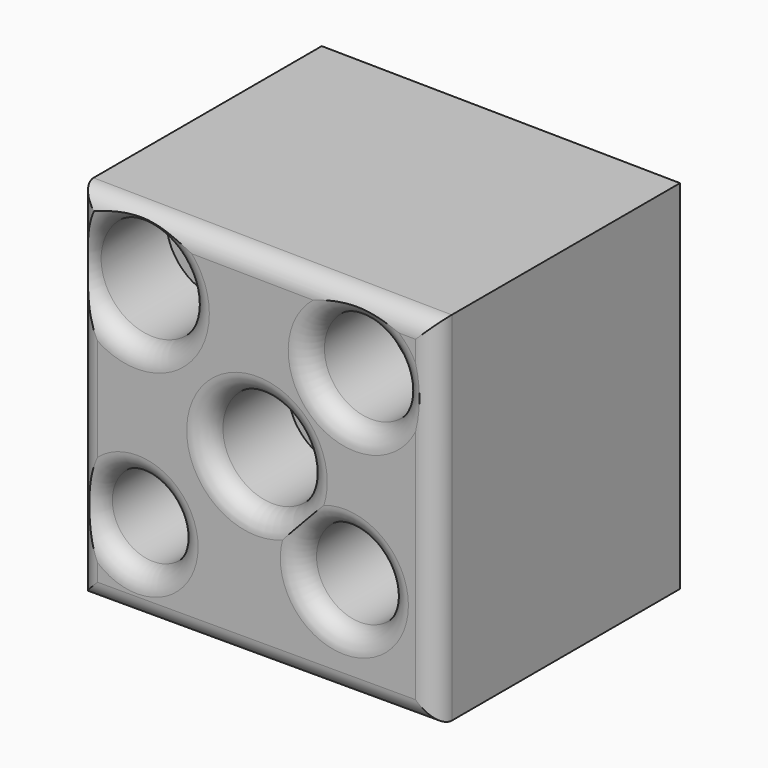
from build123d import *

# Parameters (mm, degrees)
F1_DEPTH    = 76.2
F2_R        = 13.0009566934
F2_R_2      = 11.7691858669
F2_R_3      = 12.5140273394
F2_R_4      = 10.2035026267
F2_R_5      = 10.9635179416
F4_DEPTH    = 25.4
F5_T1_DEPTH = 114.7959034965
F5_T3_DEPTH = 114.5331439546
F5_T5_DEPTH = 115.5605603925
F5_T7_DEPTH = 114.7899989954


# Not quite as in the source:
# - a fillet or chamfer that OpenCascade refuses, or shapes differently, is made with other operations: its cross-section is extruded or revolved along the edge and cut away or added


with BuildPart() as f1:
    # F0 (on Front) → F1 (new body)
    with BuildSketch(Plane.XZ):
        Polygon((56.2510117888, 48.6738197505), (-33.1341587007, 49.7012361884), (-33.1341587007, -40.4544956982), (56.2510117888, -40.4544956982), align=None)
    extrude(amount=F1_DEPTH)

    # F2 (on face) → F4 (cut)
    with BuildSketch(Plane.XZ.offset(76.2)):
        with Locations((-18.2341039181, 32.6071083546)):
            Circle(F2_R)
        with Locations((36.246843636, 30.9728365391)):
            Circle(F2_R_2)
        with Locations((11.6678411141, 5.1815295592)):
            Circle(F2_R_3)
        with Locations((-18.2341039181, -19.5480342954)):
            Circle(F2_R_4)
        with Locations((33.4707759321, -15.3220649809)):
            Circle(F2_R_5)
    extrude(amount=-F4_DEPTH, mode=Mode.SUBTRACT)

    # F5: fillet of radius 5.08 on 9 edges, made by hand

    # F5_s2 → F5_t1 (cut)
    with BuildSketch(Plane(origin=(68.3857605657, 0, -0.7860437491), x_dir=(0, 1, 0), z_dir=(-0.9999339475, 0, 0.0114935013))):
        with BuildLine():
            ThreePointArc((-71.1190343146, -49.3175258025), (-74.7121024484, -47.829228251), (-76.2004, -44.2361601171))
            Line((-76.2004, -44.2361601171), (-76.7085365685, -44.2361601171))
            ThreePointArc((-76.7085365685, -44.2361601171), (-76.7081365685, -46.7766429598), (-76.7081365685, -49.3171258025))
            Line((-76.7081365685, -49.3171258025), (-76.2, -49.8252623711))
            ThreePointArc((-76.2, -49.8252623711), (-73.6595171573, -49.8252623711), (-71.1190343146, -49.8256623711))
            Line((-71.1190343146, -49.8256623711), (-71.1190343146, -49.3175258025))
        make_face()
    extrude(amount=F5_T1_DEPTH, mode=Mode.SUBTRACT)

    # F5_s4 → F5_t3 (cut)
    with BuildSketch(Plane.XY.offset(-53.1569099511)):
        with BuildLine():
            ThreePointArc((56.2514117888, -71.1190343146), (54.7631142373, -74.7121024484), (51.1700461034, -76.2004))
            Line((51.1700461034, -76.2004), (51.1700461034, -76.7085365685))
            ThreePointArc((51.1700461034, -76.7085365685), (53.7105289461, -76.7081365685), (56.2510117888, -76.7081365685))
            Line((56.2510117888, -76.7081365685), (56.7591483574, -76.2))
            ThreePointArc((56.7591483574, -76.2), (56.7591483574, -73.6595171573), (56.7595483574, -71.1190343146))
            Line((56.7595483574, -71.1190343146), (56.2514117888, -71.1190343146))
        make_face()
    extrude(amount=F5_T3_DEPTH, mode=Mode.SUBTRACT)

    # F5_s6 → F5_t5 (cut)
    with BuildSketch(Plane.XY.offset(-53.1569099511)):
        with BuildLine():
            ThreePointArc((-33.1345587007, -71.1190343146), (-31.6462611491, -74.7121024484), (-28.0531930153, -76.2004))
            Line((-28.0531930153, -76.2004), (-28.0531930153, -76.7085365685))
            ThreePointArc((-28.0531930153, -76.7085365685), (-30.593675858, -76.7081365685), (-33.1341587007, -76.7081365685))
            Line((-33.1341587007, -76.7081365685), (-33.6422952692, -76.2))
            ThreePointArc((-33.6422952692, -76.2), (-33.6422952692, -73.6595171573), (-33.6426952692, -71.1190343146))
            Line((-33.6426952692, -71.1190343146), (-33.1345587007, -71.1190343146))
        make_face()
    extrude(amount=F5_T5_DEPTH, mode=Mode.SUBTRACT)

    # F5_s8 → F5_t7 (cut)
    with BuildSketch(Plane.YZ.offset(-45.8365729536)):
        with BuildLine():
            ThreePointArc((-76.2004, -35.3735300128), (-74.7121024484, -38.9665981466), (-71.1190343146, -40.4548956982))
            Line((-71.1190343146, -40.4548956982), (-71.1190343146, -40.9630322668))
            ThreePointArc((-71.1190343146, -40.9630322668), (-73.6595171573, -40.9626322668), (-76.2, -40.9626322668))
            Line((-76.2, -40.9626322668), (-76.7081365685, -40.4544956982))
            ThreePointArc((-76.7081365685, -40.4544956982), (-76.7081365685, -37.9140128555), (-76.7085365685, -35.3735300128))
            Line((-76.7085365685, -35.3735300128), (-76.2004, -35.3735300128))
        make_face()
    extrude(amount=F5_T7_DEPTH, mode=Mode.SUBTRACT)

    # F5_s9 → F5_t10 (revolve, cut)
    with BuildSketch(Plane.XY.offset(-19.5480342954)):
        with BuildLine():
            ThreePointArc((-2.949635606, -76.2004), (-6.5427037398, -74.7121024484), (-8.0310012914, -71.1190343146))
            Line((-8.0310012914, -71.1190343146), (-8.53913786, -71.1190343146))
            ThreePointArc((-8.53913786, -71.1190343146), (-8.53873786, -73.6595171573), (-8.53873786, -76.2))
            Line((-8.53873786, -76.2), (-8.0306012914, -76.7081365685))
            ThreePointArc((-8.0306012914, -76.7081365685), (-5.4901184487, -76.7081365685), (-2.949635606, -76.7085365685))
            Line((-2.949635606, -76.7085365685), (-2.949635606, -76.2004))
        make_face()
    revolve(axis=Axis((-18.2341039181, -76.2, -19.5480342954), (0, -1, 0)), mode=Mode.SUBTRACT)

    # F5_s11 → F5_t12 (revolve, cut)
    with BuildSketch(Plane.XY.offset(-15.3220649809)):
        with BuildLine():
            ThreePointArc((49.5152595591, -76.2004), (45.9221914252, -74.7121024484), (44.4338938736, -71.1190343146))
            Line((44.4338938736, -71.1190343146), (43.9257573051, -71.1190343146))
            ThreePointArc((43.9257573051, -71.1190343146), (43.9261573051, -73.6595171573), (43.9261573051, -76.2))
            Line((43.9261573051, -76.2), (44.4342938736, -76.7081365685))
            ThreePointArc((44.4342938736, -76.7081365685), (46.9747767164, -76.7081365685), (49.5152595591, -76.7085365685))
            Line((49.5152595591, -76.7085365685), (49.5152595591, -76.2004))
        make_face()
    revolve(axis=Axis((33.4707759321, -76.2, -15.3220649809), (0, -1, 0)), mode=Mode.SUBTRACT)

    # F5_s13 → F5_t14 (revolve, cut)
    with BuildSketch(Plane.XY.offset(5.1815295592)):
        with BuildLine():
            ThreePointArc((29.2628341389, -76.2004), (25.6697660051, -74.7121024484), (24.1814684535, -71.1190343146))
            Line((24.1814684535, -71.1190343146), (23.673331885, -71.1190343146))
            ThreePointArc((23.673331885, -71.1190343146), (23.673731885, -73.6595171573), (23.673731885, -76.2))
            Line((23.673731885, -76.2), (24.1818684535, -76.7081365685))
            ThreePointArc((24.1818684535, -76.7081365685), (26.7223512962, -76.7081365685), (29.2628341389, -76.7085365685))
            Line((29.2628341389, -76.7085365685), (29.2628341389, -76.2004))
        make_face()
    revolve(axis=Axis((11.6678411141, -76.2, 5.1815295592), (0, -1, 0)), mode=Mode.SUBTRACT)

    # F5_s15 → F5_t16 (revolve, cut)
    with BuildSketch(Plane.XY.offset(32.6071083546)):
        with BuildLine():
            ThreePointArc((-0.1521815393, -76.2004), (-3.7452496731, -74.7121024484), (-5.2335472247, -71.1190343146))
            Line((-5.2335472247, -71.1190343146), (-5.7416837932, -71.1190343146))
            ThreePointArc((-5.7416837932, -71.1190343146), (-5.7412837932, -73.6595171573), (-5.7412837932, -76.2))
            Line((-5.7412837932, -76.2), (-5.2331472247, -76.7081365685))
            ThreePointArc((-5.2331472247, -76.7081365685), (-2.692664382, -76.7081365685), (-0.1521815393, -76.7085365685))
            Line((-0.1521815393, -76.7085365685), (-0.1521815393, -76.2004))
        make_face()
    revolve(axis=Axis((-18.2341039181, -76.2, 32.6071083546), (0, -1, 0)), mode=Mode.SUBTRACT)

    # F5_s17 → F5_t18 (revolve, cut)
    with BuildSketch(Plane.XY.offset(30.9728365391)):
        with BuildLine():
            ThreePointArc((53.0969951883, -76.2004), (49.5039270545, -74.7121024484), (48.0156295029, -71.1190343146))
            Line((48.0156295029, -71.1190343146), (47.5074929344, -71.1190343146))
            ThreePointArc((47.5074929344, -71.1190343146), (47.5078929344, -73.6595171573), (47.5078929344, -76.2))
            Line((47.5078929344, -76.2), (48.0160295029, -76.7081365685))
            ThreePointArc((48.0160295029, -76.7081365685), (50.5565123456, -76.7081365685), (53.0969951883, -76.7085365685))
            Line((53.0969951883, -76.7085365685), (53.0969951883, -76.2004))
        make_face()
    revolve(axis=Axis((36.246843636, -76.2, 30.9728365391), (0, -1, 0)), mode=Mode.SUBTRACT)


solid = f1.part
